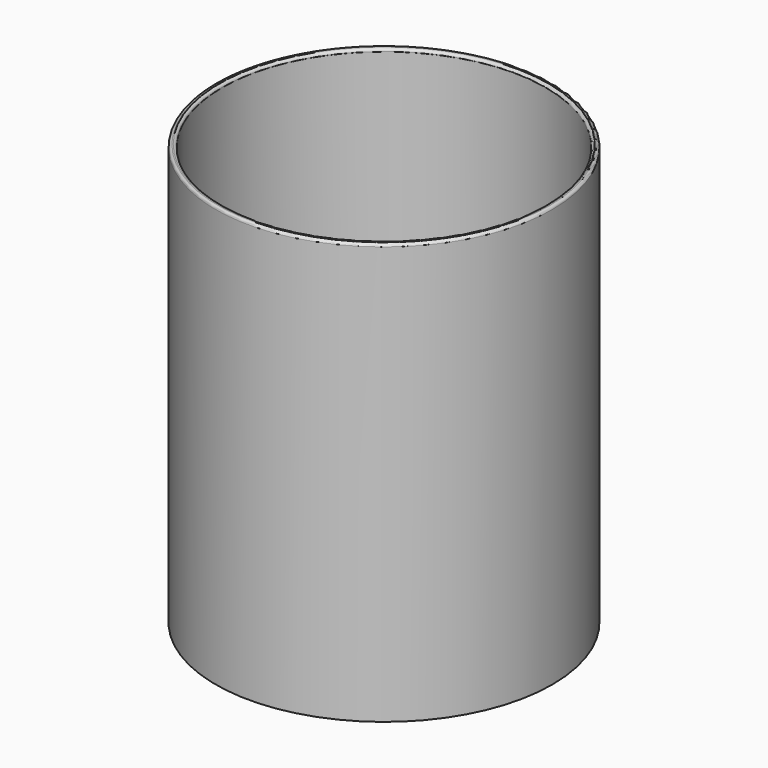
from build123d import *

# Parameters (mm, degrees)
F0_R           = 50.8
F1_DEPTH       = 127
F3_D           = 0.0254
F3_DEPTH       = 123.825
F3_CBORE_D     = 97.79
F3_CBORE_DEPTH = 123.825
F3_TIP         = 0.0076309299
F4_R           = 0.79375


with BuildPart() as f1:
    # F0 (on Top) → F1 (new body)
    with BuildSketch(Plane.XY):
        Circle(F0_R)
    extrude(amount=-F1_DEPTH)

    # F3
    with Locations(Plane.XY):
        with Locations((0, 0)):
            CounterBoreHole(F3_D / 2, F3_CBORE_D / 2, F3_CBORE_DEPTH, depth=F3_DEPTH)
            with Locations((0, 0, -(F3_DEPTH + F3_TIP / 2))):  # 118° drill point
                Cone(0, F3_D / 2, F3_TIP, mode=Mode.SUBTRACT)

    # F4
    f4_edges = [f1.edges().sort_by_distance(p)[0] for p in [
        (-50.8, 0, 0),
        (-48.895, 0, 0),
    ]]
    fillet(f4_edges, radius=F4_R)


solid = f1.part
